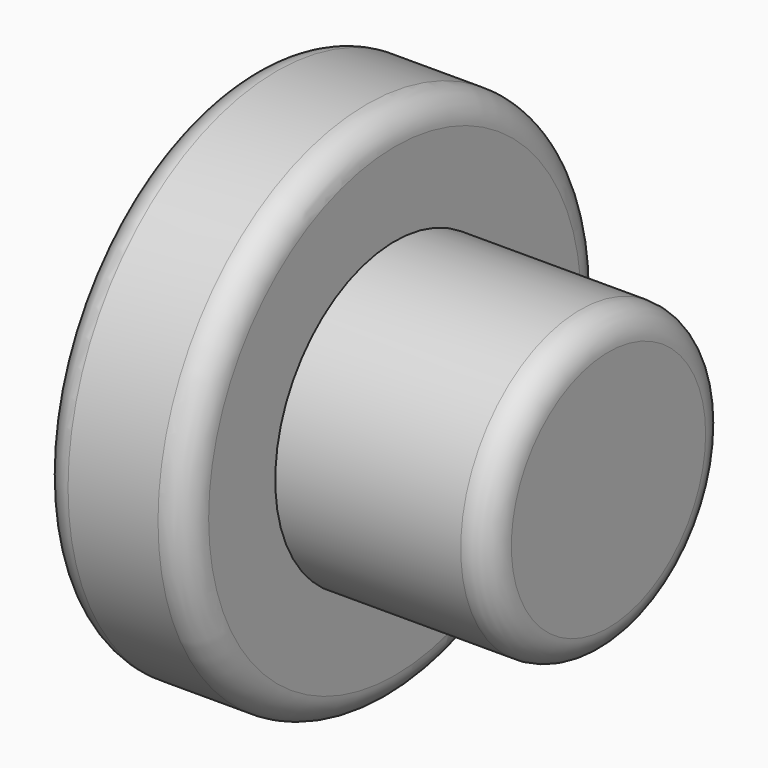
from build123d import *

# Parameters (mm, degrees)
F0_R     = 46.5439630146
F1_DEPTH = 25.4
F2_T     = -2.54
F3_R     = 26.6785648963
F4_DEPTH = 38.1
F5_T     = 2.54


# Not quite as in the source:
# - a fillet or chamfer that OpenCascade refuses, or shapes differently, is made with other operations: its cross-section is extruded or revolved along the edge and cut away or added
# - a shell that OpenCascade refuses in one call is made with other operations: the cavity is built on its own and cut out


with BuildPart() as f1:
    # F0 (on Right) → F1 (new body)
    with BuildSketch(Plane.YZ):
        Circle(F0_R)
    extrude(amount=F1_DEPTH)

    # F2
    f2_openings = [f1.faces().sort_by_distance(p)[0] for p in [
        (0, 0, 0),
    ]]
    offset(amount=F2_T, openings=f2_openings)

    # F3 (on face) → F4 (join)
    with BuildSketch(Plane.YZ.offset(25.4)):
        Circle(F3_R)
    extrude(amount=F4_DEPTH)

    # F5: shell of thickness 2.54, made by hand


with BuildPart() as f5_core1:
    # F5_t2: copy of F1
    add(f1.part)

    # the walls: a layer under each face that stays
    f5_faces = [f5_core1.faces().sort_by_distance(p)[0] for p in [
        (12.7, -46.5439630146, 0),
        (0, -43.441032147, -12.4117234706),
        (11.43, -44.0039630146, 0),
        (44.45, -26.6785648963, 0),
        (22.86, 0, 0),
        (63.5, 0, 0),
    ]]
    thicken(f5_faces, amount=-F5_T, mode=Mode.SUBTRACT)

    # F5_s3 → F5_t4 (revolve, cut)
    with BuildSketch(Plane.XY):
        Polygon((22.8346, 43.9785630146), (22.86, 46.5439630146), (25.4, 46.5439630146), (25.4, 44.0039630146), align=None)
    revolve(axis=Axis((22.86, 0, 0), (-1, 0, 0)), mode=Mode.SUBTRACT)


with BuildPart() as f1_1:
    add(f1.part)

    # what is left inside the walls is the cavity
    f5_cavity = [f5_core1.part.solids().sort_by_distance(p)[0] for p in [
        (49.106667, -24.113165, 0),
    ]]
    add(f5_cavity, mode=Mode.SUBTRACT)

    # F6: fillet of radius 5.08 on 3 edges, made by hand

    # F6_s1 → F6_t2 (revolve, cut)
    with BuildSketch(Plane.XY):
        with BuildLine():
            ThreePointArc((4.3999665546, 46.5443630146), (1.8595251638, 45.8637284922), (-0.0003463882, 44.0041630527))
            Line((-0.0003463882, 44.0041630527), (-0.4403776825, 44.258279625))
            ThreePointArc((-0.4403776825, 44.258279625), (-0.5081365685, 45.2740630337), (-0.5081365685, 46.5439630146))
            Line((-0.5081365685, 46.5439630146), (0, 47.0520995832))
            ThreePointArc((0, 47.0520995832), (2.1999832773, 47.0520995832), (4.3999665546, 47.0524995832))
            Line((4.3999665546, 47.0524995832), (4.3999665546, 46.5443630146))
        make_face()
    revolve(axis=Axis((0, 0, 0), (1, 0, 0)), mode=Mode.SUBTRACT)

    # F6_s3 → F6_t4 (revolve, cut)
    with BuildSketch(Plane.XY):
        with BuildLine():
            ThreePointArc((20.3190343146, 46.5443630146), (23.9121024484, 45.0560654631), (25.4004, 41.4629973292))
            Line((25.4004, 41.4629973292), (25.9085365685, 41.4629973292))
            ThreePointArc((25.9085365685, 41.4629973292), (25.9081365685, 44.0034801719), (25.9081365685, 46.5439630146))
            Line((25.9081365685, 46.5439630146), (25.4, 47.0520995832))
            ThreePointArc((25.4, 47.0520995832), (22.8595171573, 47.0520995832), (20.3190343146, 47.0524995832))
            Line((20.3190343146, 47.0524995832), (20.3190343146, 46.5443630146))
        make_face()
    revolve(axis=Axis((25.4, 0, 0), (1, 0, 0)), mode=Mode.SUBTRACT)

    # F6_s5 → F6_t6 (revolve, cut)
    with BuildSketch(Plane.XY):
        with BuildLine():
            ThreePointArc((58.4190343146, 26.6789648963), (62.0121024484, 25.1906673448), (63.5004, 21.5975992109))
            Line((63.5004, 21.5975992109), (64.0085365685, 21.5975992109))
            ThreePointArc((64.0085365685, 21.5975992109), (64.0081365685, 24.1380820536), (64.0081365685, 26.6785648963))
            Line((64.0081365685, 26.6785648963), (63.5, 27.1867014649))
            ThreePointArc((63.5, 27.1867014649), (60.9595171573, 27.1867014649), (58.4190343146, 27.1871014649))
            Line((58.4190343146, 27.1871014649), (58.4190343146, 26.6789648963))
        make_face()
    revolve(axis=Axis((63.5, 0, 0), (1, 0, 0)), mode=Mode.SUBTRACT)


solid = f1_1.part
